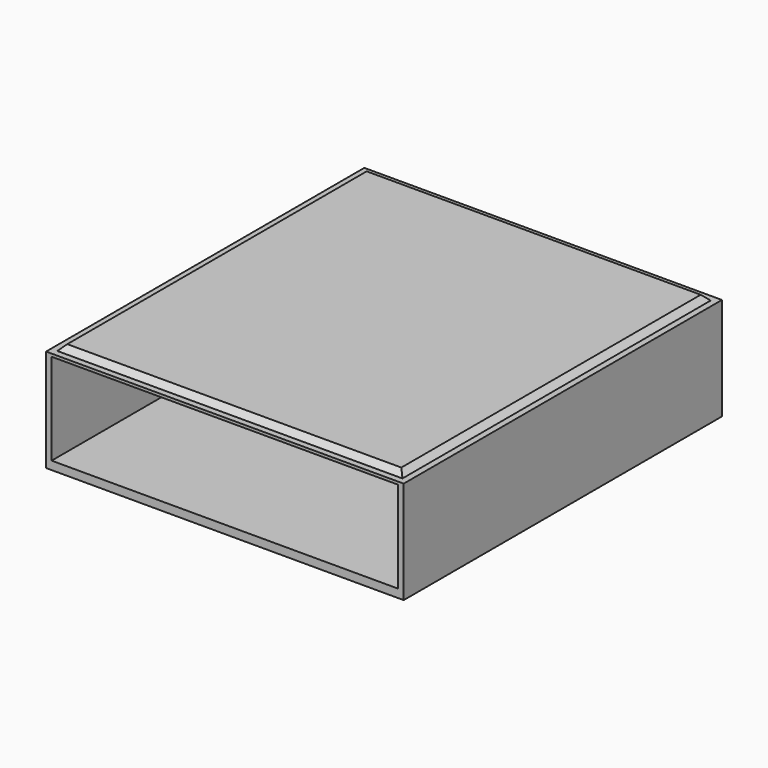
from build123d import *

# Parameters (mm, degrees)
F0_W      = 129
F0_H      = 143.5
F0_W_2    = 125
F0_H_2    = 139.5
F1_DEPTH  = 3
F2_DEPTH  = 2
F3_SIZE   = 1.99999
F5_DEPTH  = 33
F6_W      = 125
F6_H      = 141.5
F6_W_2    = 124.5
F6_H_2    = 139
F6_W_3    = 122.5
F6_H_3    = 137
F7_DEPTH  = 1
F8_DEPTH  = 3
F9_SIZE   = 1.99999
F10_DEPTH = 2
F10_TAPER = 45


# Not quite as in the source:
# - a fillet or chamfer is up to 0.001 mm smaller than in the source, because OpenCascade refuses the exact size
# - a feature names something its author has since deleted; it is built from what else it names


with BuildPart() as f1:
    # F0 (on Top) → F1 (new body)
    with BuildSketch(Plane.XY):
        Rectangle(F0_W, F0_H)
        Rectangle(F0_W_2, F0_H_2, mode=Mode.SUBTRACT)
        Rectangle(F0_W_2, F0_H_2)
    extrude(amount=F1_DEPTH)

    # F0 (on Top) → F2 (cut)
    with BuildSketch(Plane.XY):
        Rectangle(F0_W_2, F0_H_2)
    extrude(amount=F2_DEPTH, mode=Mode.SUBTRACT)

    # F3 (size 2 in the source; OpenCascade refuses exactly that, so slightly less here)
    f3_edges = [f1.edges().sort_by_distance(p)[0] for p in [
        (0, -69.75, 2),
        (62.5, 0, 2),
        (0, 69.75, 2),
        (-62.5, 0, 2),
    ]]
    chamfer(f3_edges, length=F3_SIZE)

    # F4 (on face) → F5 (join)
    with BuildSketch(Plane.XY.offset(3)):
        Polygon((-64.5, 71.75), (-64.5, -71.75), (-62.5, -71.75), (-62.5, 69.75), (62.5, 69.75), (62.5, -71.75), (64.5, -71.75), (64.5, 71.75), align=None)
    extrude(amount=F5_DEPTH)

    # F6 (on face) → F7 (join)
    with BuildSketch(Plane.XY.offset(36)):
        with Locations((0, -1)):
            Rectangle(F6_W, F6_H)
        Rectangle(F6_W_2, F6_H_2, mode=Mode.SUBTRACT)
        Rectangle(F6_W_2, F6_H_2)
        Rectangle(F6_W_3, F6_H_3, mode=Mode.SUBTRACT)
        Polygon((-64.5, 71.75), (-64.5, -71.75), (-62.5, -71.75), (-62.5, 69.75), (62.5, 69.75), (62.5, -71.75), (64.5, -71.75), (64.5, 71.75), align=None)
    extrude(amount=F7_DEPTH)

    # F6 (on face) → F8 (join)
    with BuildSketch(Plane.XY.offset(36)):
        Rectangle(F6_W_2, F6_H_2)
        Rectangle(F6_W_3, F6_H_3, mode=Mode.SUBTRACT)
        Rectangle(F6_W_3, F6_H_3)
    extrude(amount=F8_DEPTH)

    # F9 (size 2 in the source; OpenCascade refuses exactly that, so slightly less here)
    f9_edges = [f1.edges().sort_by_distance(p)[0] for p in [
        (-62.25, 0, 39),
        (0, 69.5, 39),
        (0, -69.5, 39),
        (62.25, 0, 39),
    ]]
    chamfer(f9_edges, length=F9_SIZE)

    # F6 (on face) → F10 (cut)
    with BuildSketch(Plane.XY.offset(36)):
        Rectangle(F6_W_3, F6_H_3)
    extrude(amount=F10_DEPTH, taper=F10_TAPER, mode=Mode.SUBTRACT)


solid = f1.part
